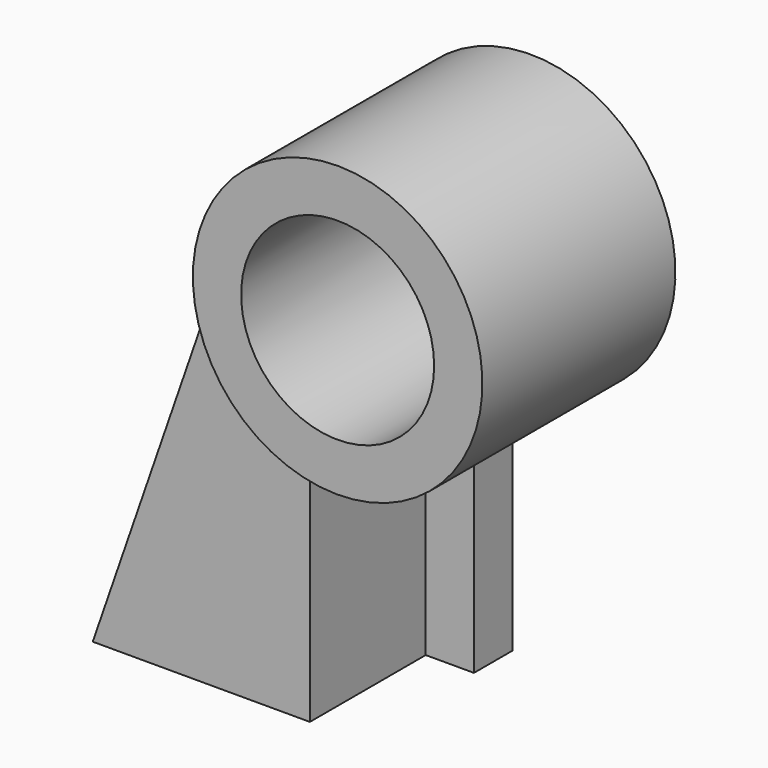
from build123d import *

# Parameters (mm, degrees)
F0_R     = 50.8
F1_DEPTH = 127
F2_DEPTH = 101.6
F4_DEPTH = 25.4


# Not quite as in the source:
# - a feature of the source that left no trace in its solid (it failed there, or was rolled back) is left out


with BuildPart() as f1:
    # F0 (on Front) → F1 (new body)
    with BuildSketch(Plane.XZ):
        with BuildLine():
            ThreePointArc((-61.2979337454, -96.1375838272), (-1.3713712696, -77.6852401135), (24.4270662546, -20.5352401135))
            ThreePointArc((24.4270662546, -20.5352401135), (24.2670376819, -15.5993769332), (23.7876241198, -10.6842454887))
            ThreePointArc((23.7876241198, -10.6842454887), (-51.7729337454, 55.6647598865), (-127.3334916106, -10.6842454887))
            ThreePointArc((-127.3334916106, -10.6842454887), (-119.2731253406, -55.8929003106), (-86.6979337454, -88.260304713))
            ThreePointArc((-86.6979337454, -88.260304713), (-74.3442320368, -93.3155705156), (-61.2979337454, -96.1375838272))
        make_face()
        with Locations((-51.7729337454, -20.5352401135)):
            Circle(F0_R, mode=Mode.SUBTRACT)
    extrude(amount=F1_DEPTH)

    # F0 (on Front) → F2 (join)
    with BuildSketch(Plane.XZ):
        with BuildLine():
            ThreePointArc((-86.6979337454, -88.260304713), (-119.2731253406, -55.8929003106), (-127.3334916106, -10.6842454887))
            Line((-127.3334916106, -10.6842454887), (-200.9979337454, -223.7352401135))
            Line((-200.9979337454, -223.7352401135), (-86.6979337454, -223.7352401135))
            Line((-86.6979337454, -223.7352401135), (-86.6979337454, -88.260304713))
        make_face()
    extrude(amount=F2_DEPTH)

    # F0 (on Front) → F4 (join)
    with BuildSketch(Plane.XZ):
        with BuildLine():
            Line((-61.2979337454, -223.7352401135), (-61.2979337454, -96.1375838272))
            ThreePointArc((-61.2979337454, -96.1375838272), (-74.3442320368, -93.3155705156), (-86.6979337454, -88.260304713))
            Line((-86.6979337454, -88.260304713), (-86.6979337454, -223.7352401135))
            Line((-86.6979337454, -223.7352401135), (-61.2979337454, -223.7352401135))
        make_face()
    extrude(amount=F4_DEPTH)


solid = f1.part
